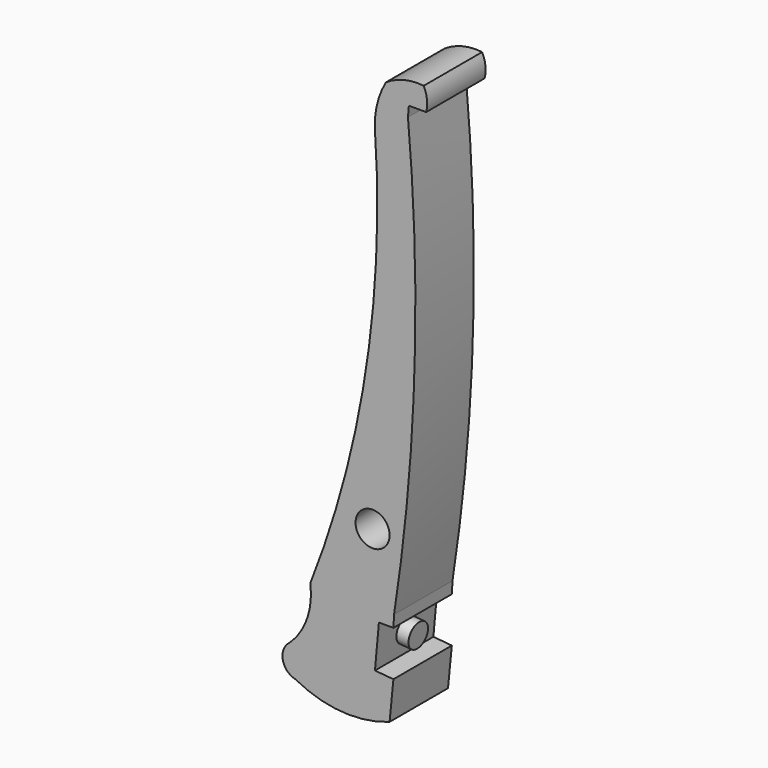
from build123d import *

# Parameters (mm, degrees)
F1_DEPTH = 3.81
F4_D     = 1.778
F5_R     = 0.6352589674
F6_DEPTH = 0.635


# Not quite as in the source:
# - a feature of the source that left no trace in its solid (it failed there, or was rolled back) is left out
# - a feature names something its author has since deleted; it is built from what else it names


with BuildPart() as f1:
    # F0 (on Front) → F1 (new body)
    with BuildSketch(Plane.XZ):
        with BuildLine():
            ThreePointArc((-31.4986416626, 9.8449740097), (-31.6959768892, 8.9855931424), (-31.0501495083, 8.3852735102))
            ThreePointArc((-31.0501495083, 8.3852735102), (-28.6350189428, 7.6831870892), (-26.1434996057, 8.026861912))
            Line((-26.1434996057, 8.026861912), (-25.9436036256, 10.0525402048))
            Line((-25.9436036256, 10.0525402048), (-26.9064083695, 10.1394830272))
            Line((-26.9064083695, 10.1394830272), (-26.7011658463, 12.4123385609))
            Line((-26.7011658463, 12.4123385609), (-25.9436036256, 12.4123385609))
            Line((-25.9436036256, 12.4123385609), (-25.9087286158, 13.0410402551))
            ThreePointArc((-25.9087286158, 13.0410402551), (-24.8435996749, 24.5554030542), (-25.1834829825, 36.1139293298))
            Line((-25.1834829825, 36.1139293298), (-25.1380671304, 36.6562315202))
            Line((-25.1380671304, 36.6562315202), (-24.2339836005, 36.6562315202))
            ThreePointArc((-24.2339836005, 36.6562315202), (-24.1923341682, 37.2519069884), (-24.3619682602, 37.8244349033))
            ThreePointArc((-24.3619682602, 37.8244349033), (-25.3896581056, 37.7581269753), (-26.3316547054, 37.3419712767))
            ThreePointArc((-26.3316547054, 37.3419712767), (-26.7797456815, 36.2582545781), (-26.9143641051, 35.0933059588))
            ThreePointArc((-26.9143641051, 35.0933059588), (-27.3654380994, 23.8788044049), (-30.282865234, 13.0410402552))
            ThreePointArc((-30.282865234, 13.0410402552), (-30.4786310467, 11.2862366956), (-31.4986416626, 9.8449740097))
        make_face()
    extrude(amount=F1_DEPTH)

    # F4 (through all)
    with Locations(Plane(origin=(0, 0, 0), x_dir=(1, 0, 0), z_dir=(0, 1, 0))):
        with Locations((-27.0313583314, -16.6009981185)):
            Hole(F4_D / 2)

    # F5 (on face) → F6 (join)
    with BuildSketch(Plane(origin=(-27.5969837191, 0, 2.4920521733), x_dir=(0, 1, 0), z_dir=(0.9959475762, 0, -0.0899356737))):
        with Locations((-1.905, 8.8195993749)):
            Circle(F5_R)
    extrude(amount=F6_DEPTH)


solid = f1.part
